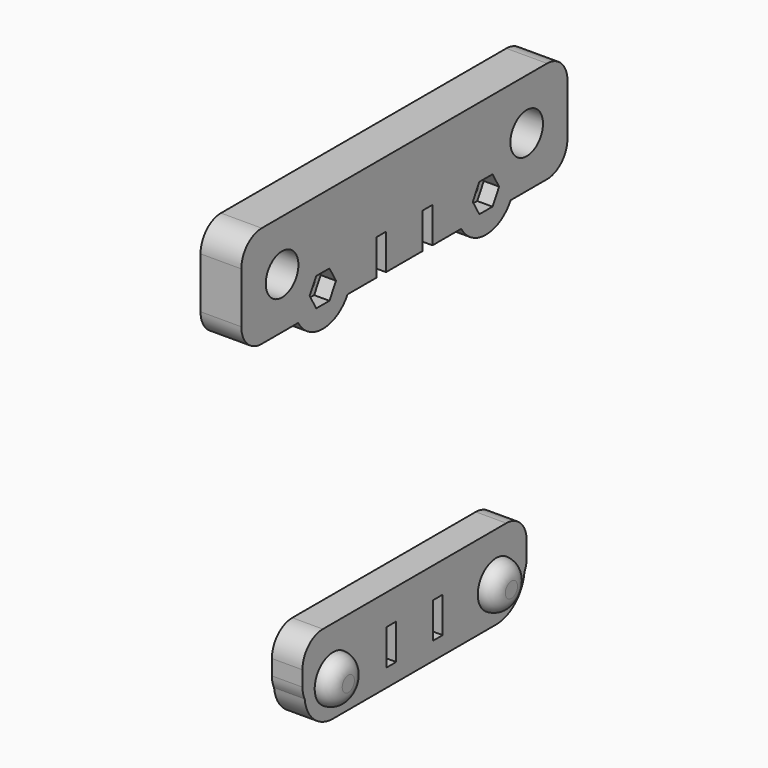
from build123d import *

# Parameters (mm, degrees)
F0_R      = 5
F0_R_2    = 4
F1_DEPTH  = 4
F2_R      = 1.4
F3_DEPTH  = 13
F4_R      = 1.8
F4_R_2    = 4
F5_DEPTH  = 4
F7_DEPTH  = 3
F8_R      = 1.9
F8_W      = 2.4
F8_H      = 7
F9_DEPTH  = 6
F11_R     = 4.5
F12_DEPTH = 3
F13_R     = 2.99999


# Not quite as in the source:
# - a fillet or chamfer is up to 0.001 mm smaller than in the source, because OpenCascade refuses the exact size


with BuildPart() as f1:
    # F0 (on Right) → F1 (new body, symmetric)
    with BuildSketch(Plane.YZ):
        with BuildLine():
            Line((-11, 25), (-35, 25))
            ThreePointArc((-35, 25), (-38.5355339059, 23.5355339059), (-40, 20))
            Line((-40, 20), (-40, -25))
            Line((-40, -25), (40, -25))
            Line((40, -25), (40, 20))
            ThreePointArc((40, 20), (38.5355339059, 23.5355339059), (35, 25))
            Line((35, 25), (11, 25))
            Line((11, 25), (11, 10))
            ThreePointArc((11, 10), (10.4142135624, 8.5857864376), (9, 8))
            Line((9, 8), (-9, 8))
            ThreePointArc((-9, 8), (-10.4142135624, 8.5857864376), (-11, 10))
            Line((-11, 10), (-11, 25))
        make_face()
        with Locations((-30, -13)):
            Circle(F0_R, mode=Mode.SUBTRACT)
        with Locations((30, -13)):
            Circle(F0_R, mode=Mode.SUBTRACT)
        with Locations((-30, 13)):
            Circle(F0_R_2, mode=Mode.SUBTRACT)
        with Locations((30, 13)):
            Circle(F0_R_2, mode=Mode.SUBTRACT)
    extrude(amount=F1_DEPTH, both=True)

    # F2 (on face) → F3 (cut)
    with BuildSketch(Plane.XY.offset(25)):
        with Locations((0, 30)):
            Circle(F2_R)
        with Locations((0, 24)):
            Circle(F2_R)
        with Locations((0, -24)):
            Circle(F2_R)
        with Locations((0, -30)):
            Circle(F2_R)
    extrude(amount=-F3_DEPTH, mode=Mode.SUBTRACT)


with BuildPart() as f5:
    # F4 (on Right) → F5 (new body, symmetric)
    with BuildSketch(Plane.YZ):
        with BuildLine():
            Line((-11, 80.1862078905), (-35, 80.1862078905))
            ThreePointArc((-35, 80.1862078905), (-38.5355339059, 78.7217417964), (-40, 75.1862078905))
            Line((-40, 75.1862078905), (-40, 65.1862078905))
            ThreePointArc((-40, 65.1862078905), (-38.5355339059, 61.6506739846), (-35, 60.1862078905))
            Line((-35, 60.1862078905), (-26.0621778265, 60.1862078905))
            ThreePointArc((-26.0621778265, 60.1862078905), (-20, 56.6862078905), (-13.9378221735, 60.1862078905))
            Line((-13.9378221735, 60.1862078905), (-6.9, 60.1862078905))
            Line((-6.9, 60.1862078905), (-6.9, 67.1862078905))
            Line((-6.9, 67.1862078905), (-4.5, 67.1862078905))
            Line((-4.5, 67.1862078905), (-4.5, 60.1862078905))
            Line((-4.5, 60.1862078905), (4.5, 60.1862078905))
            Line((4.5, 60.1862078905), (4.5, 67.1862078905))
            Line((4.5, 67.1862078905), (6.9, 67.1862078905))
            Line((6.9, 67.1862078905), (6.9, 60.1862078905))
            Line((6.9, 60.1862078905), (13.9378221735, 60.1862078905))
            ThreePointArc((13.9378221735, 60.1862078905), (20, 56.6862078905), (26.0621778265, 60.1862078905))
            Line((26.0621778265, 60.1862078905), (35, 60.1862078905))
            ThreePointArc((35, 60.1862078905), (38.5355339059, 61.6506739846), (40, 65.1862078905))
            Line((40, 65.1862078905), (40, 75.1862078905))
            ThreePointArc((40, 75.1862078905), (38.5355339059, 78.7217417964), (35, 80.1862078905))
            Line((35, 80.1862078905), (11, 80.1862078905))
            Line((11, 80.1862078905), (-11, 80.1862078905))
        make_face()
        with Locations((-20, 63.6862078905)):
            Circle(F4_R, mode=Mode.SUBTRACT)
        with Locations((20, 63.6862078905)):
            Circle(F4_R, mode=Mode.SUBTRACT)
        with Locations((-30, 70.1862078905)):
            Circle(F4_R_2, mode=Mode.SUBTRACT)
        with Locations((30, 70.1862078905)):
            Circle(F4_R_2, mode=Mode.SUBTRACT)
    extrude(amount=F5_DEPTH, both=True)

    # F6 (on face) → F7 (cut)
    with BuildSketch(Plane.YZ.offset(4)):
        Polygon((21.6165807537, 66.4862078905), (18.3834192463, 66.4862078905), (16.7668384925, 63.6862078905), (18.3834192463, 60.8862078905), (21.6165807537, 60.8862078905), (23.2331615075, 63.6862078905), align=None)
        Polygon((-18.3834192463, 66.4862078905), (-21.6165807537, 66.4862078905), (-23.2331615075, 63.6862078905), (-21.6165807537, 60.8862078905), (-18.3834192463, 60.8862078905), (-16.7668384925, 63.6862078905), align=None)
    extrude(amount=-F7_DEPTH, mode=Mode.SUBTRACT)


with BuildPart() as f9:
    # F8 (on Right) → F9 (new body)
    with BuildSketch(Plane.YZ):
        with BuildLine():
            Line((22.5, 6.5), (-22.5, 6.5))
            ThreePointArc((-22.5, 6.5), (-26.0355339059, 5.0355339059), (-27.5, 1.5))
            Line((-27.5, 1.5), (-27.5, -1.5))
            ThreePointArc((-27.5, -1.5), (-27.3626680324, -2.6638125307), (-26.9582161573, -3.7636935955))
            ThreePointArc((-26.9582161573, -3.7636935955), (-24.7038160383, -8.1840249496), (-20.085830036, -9.9994737806))
            Line((-20.085830036, -9.9994737806), (-19.9143537329, -9.9994760316))
            Line((-19.9143537329, -9.9994760316), (19.9999081087, -9.9999999994))
            ThreePointArc((19.9999081087, -9.9999999994), (24.6719110347, -8.2127964936), (26.9582161573, -3.7636935955))
            ThreePointArc((26.9582161573, -3.7636935955), (27.3626680324, -2.6638125307), (27.5, -1.5))
            Line((27.5, -1.5), (27.5, 1.5))
            ThreePointArc((27.5, 1.5), (26.0355339059, 5.0355339059), (22.5, 6.5))
        make_face()
        with Locations((-20, -3)):
            Circle(F8_R, mode=Mode.SUBTRACT)
        with Locations((-5.7, -3)):
            Rectangle(F8_W, F8_H, mode=Mode.SUBTRACT)
        with Locations((5.7, -3)):
            Rectangle(F8_W, F8_H, mode=Mode.SUBTRACT)
        with Locations((20, -3)):
            Circle(F8_R, mode=Mode.SUBTRACT)
    extrude(amount=F9_DEPTH)

    # F11 (on face) → F12 (join)
    with BuildSketch(Plane.YZ.offset(6)):
        with Locations((-20, -3)):
            Circle(F11_R)
        with Locations((20, -3)):
            Circle(F11_R)
    extrude(amount=F12_DEPTH)

    # F13 (radius 3 in the source; OpenCascade refuses exactly that, so slightly less here)
    f13_edges = [f9.edges().sort_by_distance(p)[0] for p in [
        (9, -24.5, -3),
        (9, 15.5, -3),
    ]]
    fillet(f13_edges, radius=F13_R)


solid = Compound([f5.part, f9.part])
